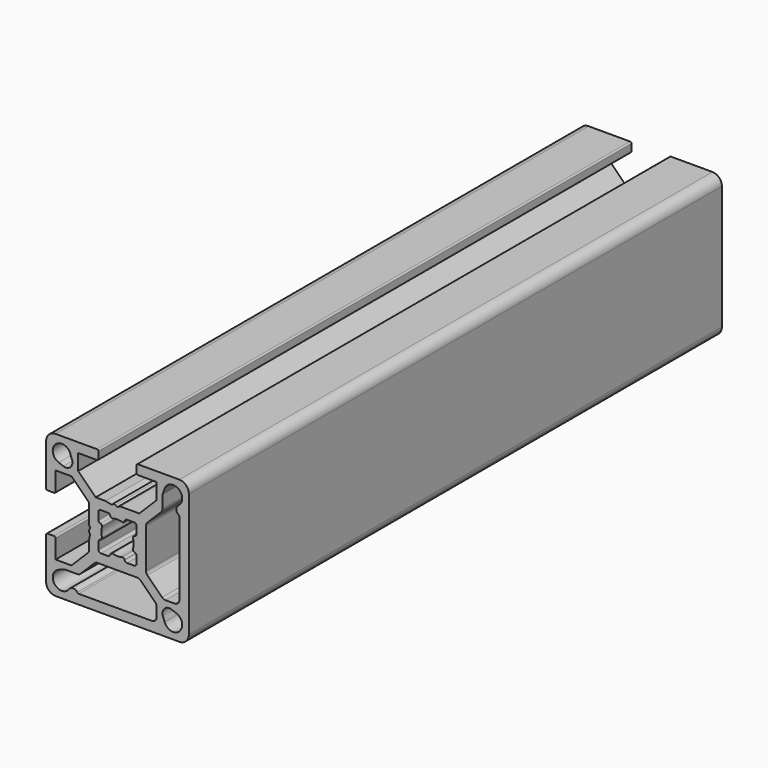
from build123d import *

# Parameters (mm, degrees)
F2_DEPTH = 70


# Not quite as in the source:
# - ends of sketch curves that miss each other by under 0.0002 mm in the source are joined


with BuildPart() as f2:
    # F1 (on Front) → F2 (new body, symmetric)
    with BuildSketch(Plane.XZ):
        with BuildLine():
            Line((-48.090856, 20.246586), (-44.140856, 20.246586))
            ThreePointArc((-44.140856, 20.246586), (-43.9287239656, 20.3344539656), (-43.840856, 20.546586))
            Line((-43.840856, 20.546586), (-43.840856, 21.946586))
            ThreePointArc((-43.840856, 21.946586), (-43.9287239656, 22.1587180344), (-44.140856, 22.246586))
            Line((-44.140856, 22.246586), (-52.840856, 22.246586))
            ThreePointArc((-52.840856, 22.246586), (-54.2550695624, 21.6607995624), (-54.840856, 20.246586))
            Line((-54.840856, 20.246586), (-54.840856, 11.546586))
            ThreePointArc((-54.840856, 11.546586), (-54.7529880344, 11.3344539656), (-54.540856, 11.246586))
            Line((-54.540856, 11.246586), (-53.140856, 11.246586))
            ThreePointArc((-53.140856, 11.246586), (-52.9287239656, 11.3344539656), (-52.840856, 11.546586))
            Line((-52.840856, 11.546586), (-52.840856, 15.496586))
            Line((-52.840856, 15.496586), (-49.50507, 15.496586))
            Line((-49.50507, 15.496586), (-45.840856, 11.832372))
            Line((-45.840856, 11.832372), (-45.840856, 7.900176))
            ThreePointArc((-45.840856, 7.900176), (-45.8238189324, 7.7707665494), (-45.7738687764, 7.6501761291))
            Line((-45.7738687764, 7.6501761291), (-45.540856, 7.246586))
            Line((-45.540856, 7.246586), (-45.773869, 6.842996))
            ThreePointArc((-45.773869, 6.842996), (-45.840856, 6.592996), (-45.7738687764, 6.3429961291))
            Line((-45.7738687764, 6.3429961291), (-45.591833, 6.0277))
            Line((-45.591833, 6.0277), (-45.840856, 4.746586))
            Line((-45.840856, 4.746586), (-45.840856, 2.6608))
            Line((-45.840856, 2.6608), (-49.50507, -1.003414))
            Line((-49.50507, -1.003414), (-52.840856, -1.003414))
            Line((-52.840856, -1.003414), (-52.840856, 2.946586))
            ThreePointArc((-52.840856, 2.946586), (-52.9287239656, 3.1587180344), (-53.140856, 3.246586))
            Line((-53.140856, 3.246586), (-54.540856, 3.246586))
            ThreePointArc((-54.540856, 3.246586), (-54.7529880344, 3.1587180344), (-54.840856, 2.946586))
            Line((-54.840856, 2.946586), (-54.840856, -5.753414))
            ThreePointArc((-54.840856, -5.753414), (-54.2550695624, -7.1676275624), (-52.840856, -7.753414))
            Line((-52.840856, -7.753414), (-26.840856, -7.753414))
            ThreePointArc((-26.840856, -7.753414), (-25.4266424376, -7.1676275624), (-24.840856, -5.753414))
            Line((-24.840856, -5.753414), (-24.840856, 20.246586))
            ThreePointArc((-24.840856, 20.246586), (-25.4266424376, 21.6607995624), (-26.840856, 22.246586))
            Line((-26.840856, 22.246586), (-35.540856, 22.246586))
            ThreePointArc((-35.540856, 22.246586), (-35.7529880344, 22.1587180344), (-35.840856, 21.946586))
            Line((-35.840856, 21.946586), (-35.840856, 20.546586))
            ThreePointArc((-35.840856, 20.546586), (-35.7529880344, 20.3344539656), (-35.540856, 20.246586))
            Line((-35.540856, 20.246586), (-31.590856, 20.246586))
            Line((-31.590856, 20.246586), (-31.590856, 16.9108))
            Line((-31.590856, 16.9108), (-35.25507, 13.246586))
            Line((-35.25507, 13.246586), (-39.187266, 13.246586))
            ThreePointArc((-39.187266, 13.246586), (-39.3166754506, 13.2295489324), (-39.4372658709, 13.1795987764))
            Line((-39.4372658709, 13.1795987764), (-39.840856, 12.946586))
            Line((-39.840856, 12.946586), (-40.244446, 13.179599))
            ThreePointArc((-40.244446, 13.179599), (-40.494446, 13.246586), (-40.7444458709, 13.1795987764))
            Line((-40.7444458709, 13.1795987764), (-41.059742, 12.997563))
            Line((-41.059742, 12.997563), (-42.340856, 13.246586))
            Line((-42.340856, 13.246586), (-44.426642, 13.246586))
            Line((-44.426642, 13.246586), (-48.090856, 16.9108))
            Line((-48.090856, 16.9108), (-48.090856, 20.246586))
        make_face()
        with BuildLine():
            ThreePointArc((-48.030175, -5.753414), (-48.180175082, -5.7132215738), (-48.2899827159, -5.6034138359))
            ThreePointArc((-48.2899827159, -5.6034138359), (-49.1151948384, -5.1042472042), (-49.9783690315, -5.5344479782))
            ThreePointArc((-49.9783690315, -5.5344479782), (-53.0449723505, -5.6142903949), (-52.1906940253, -2.6679979306))
            Line((-52.1906940253, -2.6679979306), (-50.91426, -2.203414))
            Line((-50.91426, -2.203414), (-48.290856, -2.203414))
            ThreePointArc((-48.290856, -2.203414), (-47.9081725676, -2.1272935325), (-47.5837492188, -1.9105207812))
            Line((-47.5837492188, -1.9105207812), (-44.719536, 0.953693))
            ThreePointArc((-44.719536, 0.953693), (-44.3951124324, 1.1704655325), (-44.012429, 1.246586))
            Line((-44.012429, 1.246586), (-35.669283, 1.246586))
            ThreePointArc((-35.669283, 1.246586), (-35.2865995676, 1.1704655325), (-34.9621762188, 0.9536927812))
            Line((-34.9621762188, 0.9536927812), (-31.883749, -2.124734))
            ThreePointArc((-31.883749, -2.124734), (-31.6669764675, -2.4491575676), (-31.590856, -2.831841))
            Line((-31.590856, -2.831841), (-31.590856, -4.753414))
            ThreePointArc((-31.590856, -4.753414), (-31.8837492188, -5.4605207812), (-32.590856, -5.753414))
            Line((-32.590856, -5.753414), (-48.030175, -5.753414))
        make_face(mode=Mode.SUBTRACT)
        with BuildLine():
            ThreePointArc((-30.2930043339, -4.0956641215), (-29.9673844937, -2.6268855063), (-28.4986058785, -2.3012656661))
            Line((-28.4986058785, -2.3012656661), (-27.491018, -2.667998))
            ThreePointArc((-27.491018, -2.667998), (-26.7973531157, -5.7969168843), (-29.9262720694, -5.1032520253))
            Line((-29.9262720694, -5.1032520253), (-30.2930043339, -4.0956641215))
        make_face(mode=Mode.SUBTRACT)
        with BuildLine():
            ThreePointArc((-36.5876690145, 8.2349049956), (-36.440856, 7.246586), (-36.5876690145, 6.2582670044))
            ThreePointArc((-36.5876690145, 6.2582670044), (-36.5433888407, 5.9288023569), (-36.2653470651, 5.7465855742))
            ThreePointArc((-36.2653470651, 5.7465855742), (-35.9615444769, 5.5780848975), (-35.840856, 5.25232))
            Line((-35.840856, 5.25232), (-35.840856, 3.746586))
            ThreePointArc((-35.840856, 3.746586), (-35.9873026094, 3.3930326094), (-36.340856, 3.246586))
            Line((-36.340856, 3.246586), (-37.84659, 3.246586))
            ThreePointArc((-37.84659, 3.246586), (-38.1723548975, 3.3672744769), (-38.3408555178, 3.6710770737))
            ThreePointArc((-38.3408555178, 3.6710770737), (-38.5230723569, 3.9491188407), (-38.8525409519, 3.9933978415))
            ThreePointArc((-38.8525409519, 3.9933978415), (-39.840856, 3.846586), (-40.8291749956, 3.9933990145))
            ThreePointArc((-40.8291749956, 3.9933990145), (-41.1586396431, 3.9491188407), (-41.3408564258, 3.6710770651))
            ThreePointArc((-41.3408564258, 3.6710770651), (-41.5093571025, 3.3672744769), (-41.835122, 3.246586))
            Line((-41.835122, 3.246586), (-43.340856, 3.246586))
            ThreePointArc((-43.340856, 3.246586), (-43.6944093906, 3.3930326094), (-43.840856, 3.746586))
            Line((-43.840856, 3.746586), (-43.840856, 5.25232))
            ThreePointArc((-43.840856, 5.25232), (-43.7201675231, 5.5780848975), (-43.4163649263, 5.7465855178))
            ThreePointArc((-43.4163649263, 5.7465855178), (-43.1383231593, 5.9288023569), (-43.0940441585, 6.2582709519))
            ThreePointArc((-43.0940441585, 6.2582709519), (-43.240856, 7.246586), (-43.0940429855, 8.2349049956))
            ThreePointArc((-43.0940429855, 8.2349049956), (-43.1383231593, 8.5643696431), (-43.4163649349, 8.7465864258))
            ThreePointArc((-43.4163649349, 8.7465864258), (-43.7201675231, 8.9150871025), (-43.840856, 9.240852))
            Line((-43.840856, 9.240852), (-43.840856, 10.746586))
            ThreePointArc((-43.840856, 10.746586), (-43.6944093906, 11.1001393906), (-43.340856, 11.246586))
            Line((-43.340856, 11.246586), (-41.835122, 11.246586))
            ThreePointArc((-41.835122, 11.246586), (-41.5093571025, 11.1258975231), (-41.3408564822, 10.8220949263))
            ThreePointArc((-41.3408564822, 10.8220949263), (-41.1586396431, 10.5440531593), (-40.8291710481, 10.4997741585))
            ThreePointArc((-40.8291710481, 10.4997741585), (-39.840856, 10.646586), (-38.8525370044, 10.4997729855))
            ThreePointArc((-38.8525370044, 10.4997729855), (-38.5230723569, 10.5440531593), (-38.3408555742, 10.8220949349))
            ThreePointArc((-38.3408555742, 10.8220949349), (-38.1723548975, 11.1258975231), (-37.84659, 11.246586))
            Line((-37.84659, 11.246586), (-36.340856, 11.246586))
            ThreePointArc((-36.340856, 11.246586), (-35.9873026094, 11.1001393906), (-35.840856, 10.746586))
            Line((-35.840856, 10.746586), (-35.840856, 9.240852))
            ThreePointArc((-35.840856, 9.240852), (-35.9615444769, 8.9150871025), (-36.2653470737, 8.7465864822))
            ThreePointArc((-36.2653470737, 8.7465864822), (-36.5433888407, 8.5643696431), (-36.5876690145, 8.2349049956))
        make_face(mode=Mode.SUBTRACT)
        with BuildLine():
            ThreePointArc((-49.3887076661, 18.5888361215), (-49.7143275063, 17.1200575063), (-51.1831061215, 16.7944376661))
            Line((-51.1831061215, 16.7944376661), (-52.190694, 17.16117))
            ThreePointArc((-52.190694, 17.16117), (-52.8843588843, 20.2900888843), (-49.7554399306, 19.5964240253))
            Line((-49.7554399306, 19.5964240253), (-49.3887076661, 18.5888361215))
        make_face(mode=Mode.SUBTRACT)
        with BuildLine():
            ThreePointArc((-33.5479627812, 2.3679062188), (-33.7647355325, 2.6923295676), (-33.840856, 3.075013))
            Line((-33.840856, 3.075013), (-33.840856, 11.418159))
            ThreePointArc((-33.840856, 11.418159), (-33.7647355325, 11.8008424324), (-33.5479627812, 12.1252657812))
            Line((-33.5479627812, 12.1252657812), (-30.683749, 14.989479))
            ThreePointArc((-30.683749, 14.989479), (-30.4669764675, 15.3139025676), (-30.390856, 15.696586))
            Line((-30.390856, 15.696586), (-30.390856, 18.31999))
            Line((-30.390856, 18.31999), (-29.926272, 19.596424))
            ThreePointArc((-29.926272, 19.596424), (-26.9799796051, 20.4507023505), (-27.0598220201, 17.3840990291))
            ThreePointArc((-27.0598220201, 17.3840990291), (-27.4900227958, 16.5209248384), (-26.9908561748, 15.6957126972))
            ThreePointArc((-26.9908561748, 15.6957126972), (-26.8810484262, 15.585905082), (-26.840856, 15.435905))
            Line((-26.840856, 15.435905), (-26.840856, -0.003414))
            ThreePointArc((-26.840856, -0.003414), (-27.1337492188, -0.7105207812), (-27.840856, -1.003414))
            Line((-27.840856, -1.003414), (-29.762429, -1.003414))
            ThreePointArc((-29.762429, -1.003414), (-30.1451124324, -0.9272935325), (-30.4695357812, -0.7105207812))
            Line((-30.4695357812, -0.7105207812), (-33.5479627812, 2.3679062188))
        make_face(mode=Mode.SUBTRACT)
    extrude(amount=F2_DEPTH, both=True)


solid = f2.part
